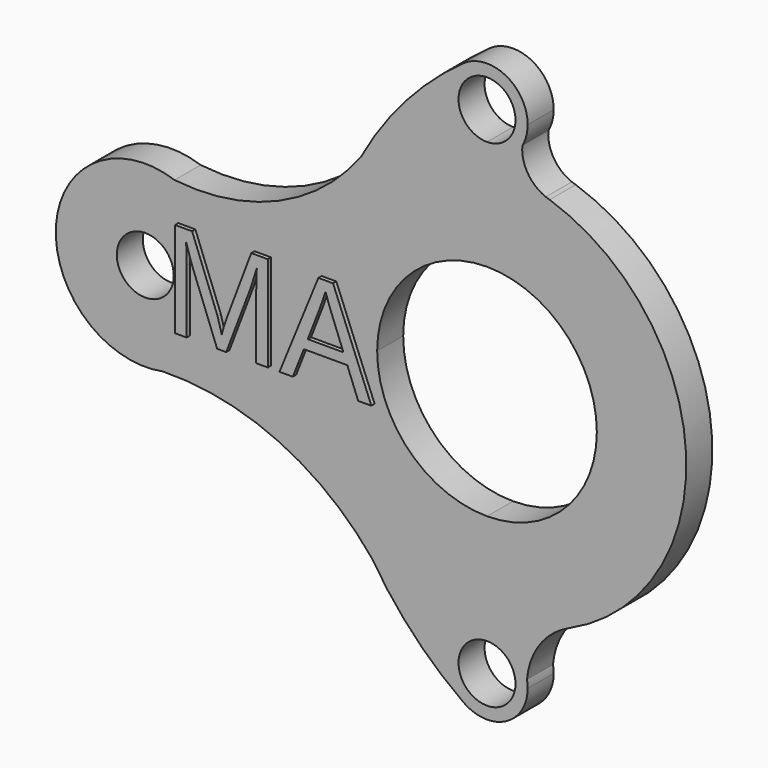
from build123d import *

# Parameters (mm, degrees)
F0_R         = 7
F1_DEPTH     = 8
F2_TEXT_SIZE = 34.065829176
F3_DEPTH     = 1


# Not quite as in the source:
# - Text() gives the source's letters only with a copy of the font that has no kerning and outlines rounded to 1/6400 em; it was checked with that copy


with BuildPart() as f1:
    # F0 (on Front) → F1 (new body)
    with BuildSketch(Plane.XZ):
        with BuildLine():
            ThreePointArc((-27, 0), (-19.091883092, 19.091883092), (0, 27))
            Line((0, 27), (0, 51))
            ThreePointArc((0, 51), (-9.5219045714, 57.9449495367), (-5.8179797945, 69.1333333333))
            ThreePointArc((-5.8179797945, 69.1333333333), (-19.9608636248, 56.3966790211), (-30.9152166607, 40.8324355227))
            ThreePointArc((-30.9152166607, 40.8324355227), (-51.1602201406, 24.6309653624), (-76.8037971755, 20.7897730846))
            ThreePointArc((-76.8037971755, 20.7897730846), (-105.9472499676, 1.5225698211), (-79.7434583893, -21.5842964564))
            ThreePointArc((-79.7434583893, -21.5842964564), (-51.217918681, -27.4652465845), (-28.2448460695, -45.3685961272))
            ThreePointArc((-28.2448460695, -45.3685961272), (-18.1841288439, -58.3387867998), (-5.8179797945, -69.1333333333))
            ThreePointArc((-5.8179797945, -69.1333333333), (-9.5219045714, -57.9449495367), (0, -51))
            Line((0, -51), (0, -27))
            ThreePointArc((0, -27), (-19.091883092, -19.091883092), (-27, 0))
        make_face()
        with Locations((-84, 0)):
            Circle(F0_R, mode=Mode.SUBTRACT)
        with BuildLine():
            ThreePointArc((0, 27), (19.091883092, 19.091883092), (27, 0))
            ThreePointArc((27, 0), (19.091883092, -19.091883092), (0, -27))
            Line((0, -27), (0, -51))
            ThreePointArc((0, -51), (6.3791141744, -53.298902523), (9.8252360148, -59.13861953))
            ThreePointArc((9.8252360148, -59.13861953), (12.9730446881, -50.5463629958), (20.0288679811, -44.7196203852))
            ThreePointArc((20.0288679811, -44.7196203852), (20.0819610634, -44.6956590858), (20.1351336519, -44.6718747404))
            ThreePointArc((20.1351336519, -44.6718747404), (48.9344682017, 2.5333420244), (15.4145211866, 46.5122837172))
            ThreePointArc((15.4145211866, 46.5122837172), (14.9373653686, 46.6507387959), (14.4685319245, 46.8151853991))
            ThreePointArc((14.4685319245, 46.8151853991), (10.0322377755, 50.4602904425), (8.6840861355, 56.041507488))
            ThreePointArc((8.6840861355, 56.041507488), (5.0207108501, 52.3517364425), (0, 51))
            Line((0, 51), (0, 27))
        make_face()
        with BuildLine():
            ThreePointArc((9.8252360148, -59.13861953), (6.3791141744, -53.298902523), (0, -51))
            ThreePointArc((0, -51), (-9.5219045714, -57.9449495367), (-5.8179797945, -69.1333333333))
            ThreePointArc((-5.8179797945, -69.1333333333), (4.5727563928, -69.8932501917), (10, -61))
            ThreePointArc((10, -61), (9.9562131392, -60.0652166421), (9.8252360148, -59.13861953))
        make_face()
        with BuildLine():
            ThreePointArc((7, -61), (-4.9497474683, -65.9497474683), (0, -54))
            ThreePointArc((0, -54), (4.9497474683, -56.0502525317), (7, -61))
        make_face(mode=Mode.SUBTRACT)
        with BuildLine():
            ThreePointArc((-5.8179797945, 69.1333333333), (-9.5219045714, 57.9449495367), (0, 51))
            ThreePointArc((0, 51), (5.0207108501, 52.3517364425), (8.6840861355, 56.041507488))
            ThreePointArc((8.6840861355, 56.041507488), (9.6654244955, 58.4349328815), (10, 61))
            ThreePointArc((10, 61), (4.5727563928, 69.8932501917), (-5.8179797945, 69.1333333333))
        make_face()
        with BuildLine():
            ThreePointArc((7, 61), (4.9497474683, 56.0502525317), (0, 54))
            ThreePointArc((0, 54), (-4.9497474683, 65.9497474683), (7, 61))
        make_face(mode=Mode.SUBTRACT)
    extrude(amount=F1_DEPTH)

    # F2 (on face) → F3 (join)
    with BuildSketch(Plane.XZ.offset(8)):
        with Locations((-78.6569835618, -11.6631016135)):
            Text('MA', F2_TEXT_SIZE, font='Arimo', text_align=(TextAlign.LEFT, TextAlign.BOTTOM))
    extrude(amount=F3_DEPTH)


solid = f1.part
